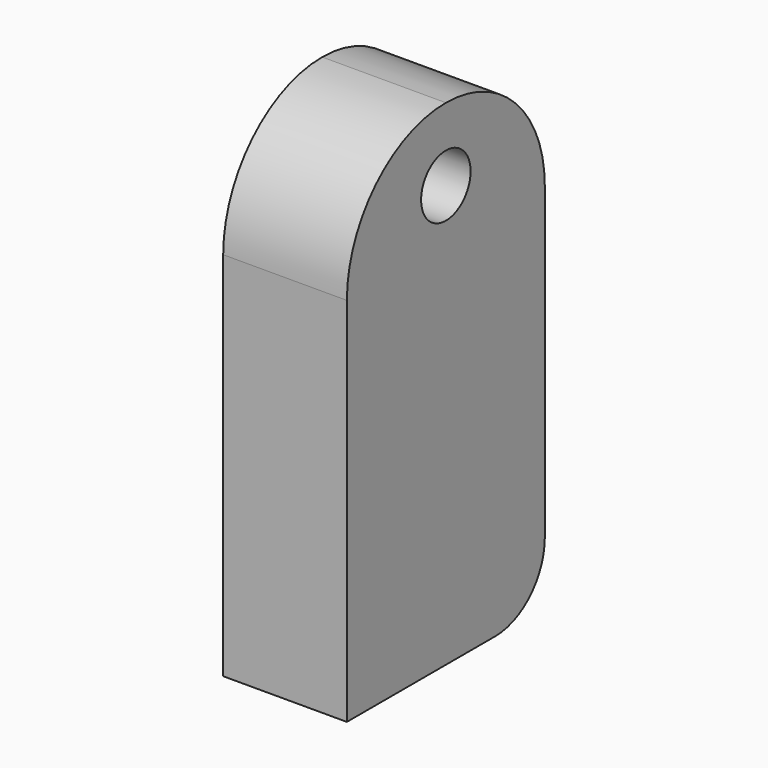
from build123d import *

# Parameters (mm, degrees)
F0_W     = 12.7
F0_H     = 50.8
F1_DEPTH = 25.4
F2_R     = 3.175
F3_DEPTH = 25.4
F4_R     = 12.7
F5_R     = 12.69999
F6_R     = 6.35


# Not quite as in the source:
# - a fillet or chamfer is up to 0.001 mm smaller than in the source, because OpenCascade refuses the exact size


with BuildPart() as f1:
    # F0 (on Front) → F1 (new body)
    with BuildSketch(Plane.XZ):
        Rectangle(F0_W, F0_H)
    extrude(amount=F1_DEPTH)

    # F2 (on face) → F3 (cut)
    with BuildSketch(Plane.YZ.offset(6.35)):
        with Locations((-12.7, 17.9132968187)):
            Circle(F2_R)
    extrude(amount=-F3_DEPTH, mode=Mode.SUBTRACT)

    # F4
    f4_edges = [f1.edges().sort_by_distance(p)[0] for p in [
        (0, -25.4, 25.4),
    ]]
    fillet(f4_edges, radius=F4_R)

    # F5 (radius 12.7 in the source; OpenCascade refuses exactly that, so slightly less here)
    f5_edges = [f1.edges().sort_by_distance(p)[0] for p in [
        (0, 0, 25.4),
    ]]
    fillet(f5_edges, radius=F5_R)

    # F6
    f6_edges = [f1.edges().sort_by_distance(p)[0] for p in [
        (0, 0, -25.4),
    ]]
    fillet(f6_edges, radius=F6_R)


solid = f1.part
